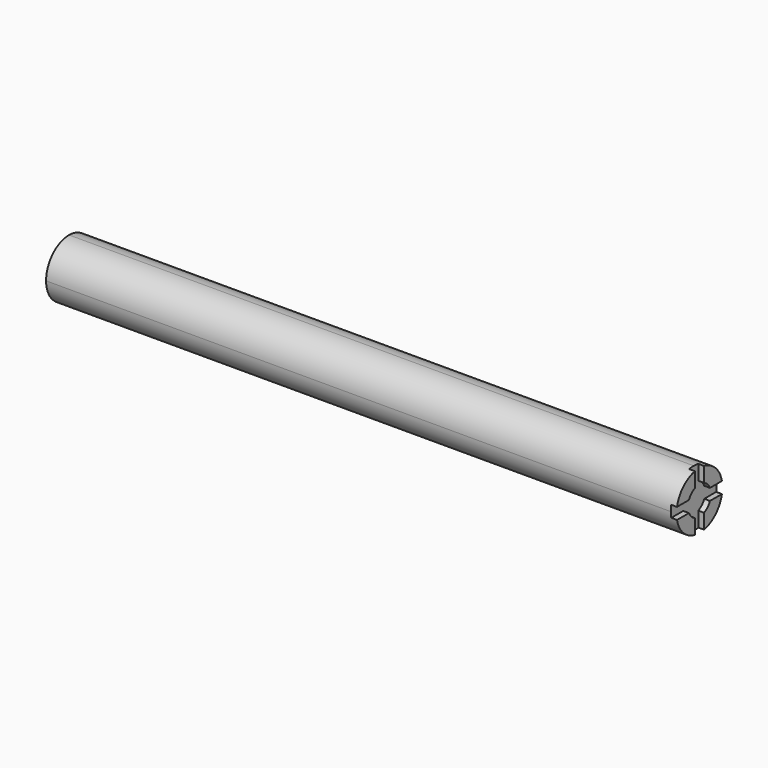
from build123d import *

# Parameters (mm, degrees)
F0_W        = 25.4
F0_H        = 25.4
F1_DEPTH    = 279.4
F3_DEPTH    = 2.54
F4_T1_DEPTH = 342.9


# Not quite as in the source:
# - a fillet or chamfer that OpenCascade refuses, or shapes differently, is made with other operations: its cross-section is extruded or revolved along the edge and cut away or added


with BuildPart() as f1:
    # F0 (on Right) → F1 (new body)
    with BuildSketch(Plane.YZ):
        with Locations((12.7, 12.7)):
            Rectangle(F0_W, F0_H)
    extrude(amount=F1_DEPTH)

    # F2 (on face) → F3 (cut)
    with BuildSketch(Plane.YZ.offset(279.4)):
        with BuildLine():
            Line((15.24, 25.4), (12.7, 25.4))
            Line((12.7, 25.4), (12.7, 19.05))
            ThreePointArc((12.7, 19.05), (13.9973662374, 18.9160550871), (15.24, 18.5198711326))
            Line((15.24, 18.5198711326), (15.24, 25.4))
        make_face()
        with BuildLine():
            Line((12.7, 19.05), (12.7, 25.4))
            Line((12.7, 25.4), (10.16, 25.4))
            Line((10.16, 25.4), (10.16, 18.5198711326))
            ThreePointArc((10.16, 18.5198711326), (11.4026337626, 18.9160550871), (12.7, 19.05))
        make_face()
        with BuildLine():
            ThreePointArc((15.24, 18.5198711326), (13.9973662374, 18.9160550871), (12.7, 19.05))
            Line((12.7, 19.05), (12.7, 18.5198711326))
            Line((12.7, 18.5198711326), (15.24, 18.5198711326))
        make_face()
        with BuildLine():
            Line((12.7, 18.5198711326), (12.7, 19.05))
            ThreePointArc((12.7, 19.05), (11.4026337626, 18.9160550871), (10.16, 18.5198711326))
            Line((10.16, 18.5198711326), (12.7, 18.5198711326))
        make_face()
        with BuildLine():
            Line((15.24, 18.5198711326), (12.7, 18.5198711326))
            Line((12.7, 18.5198711326), (10.16, 18.5198711326))
            ThreePointArc((10.16, 18.5198711326), (8.2098719395, 17.1901280605), (6.8801288674, 15.24))
            ThreePointArc((6.8801288674, 15.24), (6.35, 12.7), (6.8801288674, 10.16))
            ThreePointArc((6.8801288674, 10.16), (8.2098719395, 8.2098719395), (10.16, 6.8801288674))
            Line((10.16, 6.8801288674), (15.24, 6.8801288674))
            ThreePointArc((15.24, 6.8801288674), (17.1901280605, 8.2098719395), (18.5198711326, 10.16))
            ThreePointArc((18.5198711326, 10.16), (18.9160550871, 11.4026337626), (19.05, 12.7))
            ThreePointArc((19.05, 12.7), (18.9160550871, 13.9973662374), (18.5198711326, 15.24))
            ThreePointArc((18.5198711326, 15.24), (17.1901280605, 17.1901280605), (15.24, 18.5198711326))
        make_face()
        with BuildLine():
            Line((25.4, 15.24), (18.5198711326, 15.24))
            ThreePointArc((18.5198711326, 15.24), (18.9160550871, 13.9973662374), (19.05, 12.7))
            ThreePointArc((19.05, 12.7), (18.9160550871, 11.4026337626), (18.5198711326, 10.16))
            Line((18.5198711326, 10.16), (25.4, 10.16))
            Line((25.4, 10.16), (25.4, 15.24))
        make_face()
        with BuildLine():
            ThreePointArc((6.8801288674, 10.16), (6.35, 12.7), (6.8801288674, 15.24))
            Line((6.8801288674, 15.24), (0, 15.24))
            Line((0, 15.24), (0, 10.16))
            Line((0, 10.16), (6.8801288674, 10.16))
        make_face()
        with BuildLine():
            Line((15.24, 6.8801288674), (10.16, 6.8801288674))
            ThreePointArc((10.16, 6.8801288674), (12.7, 6.35), (15.24, 6.8801288674))
        make_face()
        with BuildLine():
            ThreePointArc((15.24, 6.8801288674), (12.7, 6.35), (10.16, 6.8801288674))
            Line((10.16, 6.8801288674), (10.16, 0))
            Line((10.16, 0), (15.24, 0))
            Line((15.24, 0), (15.24, 6.8801288674))
        make_face()
    extrude(amount=-F3_DEPTH, mode=Mode.SUBTRACT)

    # F4: fillet of radius 12.7 on 4 edges, made by hand

    # F4_s2 → F4_t1 (cut)
    with BuildSketch(Plane.YZ.offset(-31.75)):
        with BuildLine():
            ThreePointArc((12.7, 25.4), (21.6802561211, 21.6802561211), (25.4, 12.7))
            Line((25.4, 12.7), (25.4, 25.4))
            Line((25.4, 25.4), (12.7, 25.4))
        make_face()
        with BuildLine():
            ThreePointArc((12.7, 0), (21.6802561211, 3.7197438789), (25.4, 12.7))
            Line((25.4, 12.7), (25.4, 0))
            Line((25.4, 0), (12.7, 0))
        make_face()
        with BuildLine():
            ThreePointArc((0, 12.7), (3.7197438789, 21.6802561211), (12.7, 25.4))
            Line((12.7, 25.4), (0, 25.4))
            Line((0, 25.4), (0, 12.7))
        make_face()
        with BuildLine():
            ThreePointArc((0, 12.7), (3.7197438789, 3.7197438789), (12.7, 0))
            Line((12.7, 0), (0, 0))
            Line((0, 0), (0, 12.7))
        make_face()
    extrude(amount=F4_T1_DEPTH, mode=Mode.SUBTRACT)


solid = f1.part
